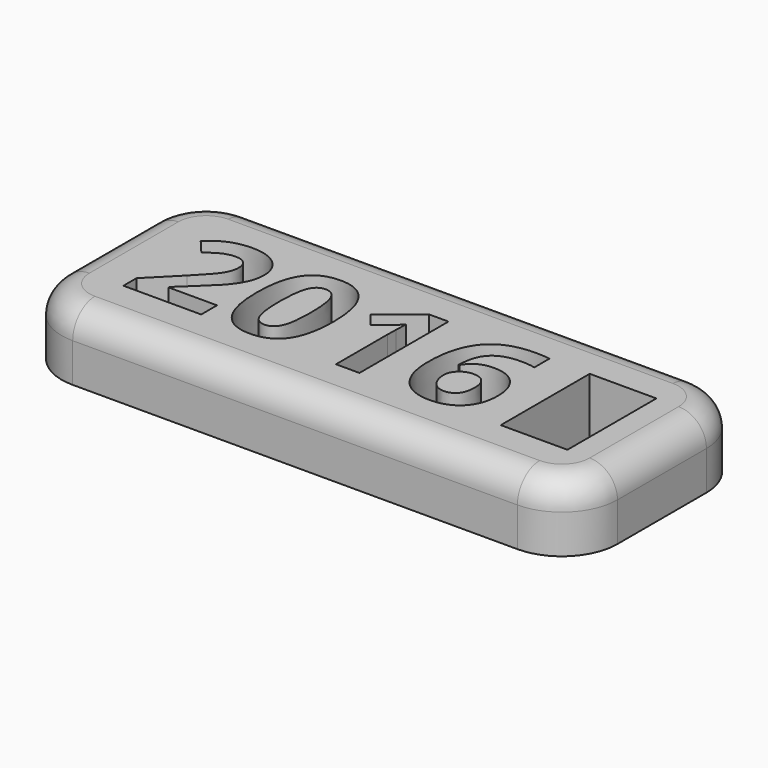
from build123d import *

# Parameters (mm, degrees)
F1_DEPTH     = 12
F2_DEPTH     = 1
F3_R         = 10
F4_R         = 5
F5_TEXT_SIZE = 28.0366295224
F6_DEPTH     = 10


# Not quite as in the source:
# - Text() gives the source's letters only with a copy of the font that has no kerning and outlines rounded to 1/6400 em; it was checked with that copy


with BuildPart() as f1:
    # F0 (on Top) → F1 (new body)
    with BuildSketch(Plane.XY):
        Polygon((-50, -20), (50, -20), (50, 0), (50, 20), (-50, 20), align=None)
        Polygon((41, 10), (41, 0), (41, -10), (29, -10), (29, 10), align=None, mode=Mode.SUBTRACT)
    extrude(amount=F1_DEPTH)

    # F0 (on Top) → F2 (join)
    with BuildSketch(Plane.XY):
        Polygon((41, -10), (41, 0), (41, 10), (29, 10), (29, -10), align=None)
    extrude(amount=F2_DEPTH)

    # F3
    f3_edges = [f1.edges().sort_by_distance(p)[0] for p in [
        (50, -20, 6),
        (50, 20, 6),
        (-50, 20, 6),
        (-50, -20, 6),
    ]]
    fillet(f3_edges, radius=F3_R)

    # F4
    f4_edges = [f1.edges().sort_by_distance(p)[0] for p in [
        (0, 20, 12),
    ]]
    fillet(f4_edges, radius=F4_R)

    # F5 (on face) → F6 (cut)
    with BuildSketch(Plane.XY.offset(12)):
        with Locations((-40, -10)):
            Text('2016', F5_TEXT_SIZE, font='Open Sans', font_style=FontStyle.BOLD, text_align=(TextAlign.LEFT, TextAlign.BOTTOM))
    extrude(amount=-F6_DEPTH, mode=Mode.SUBTRACT)


solid = f1.part
